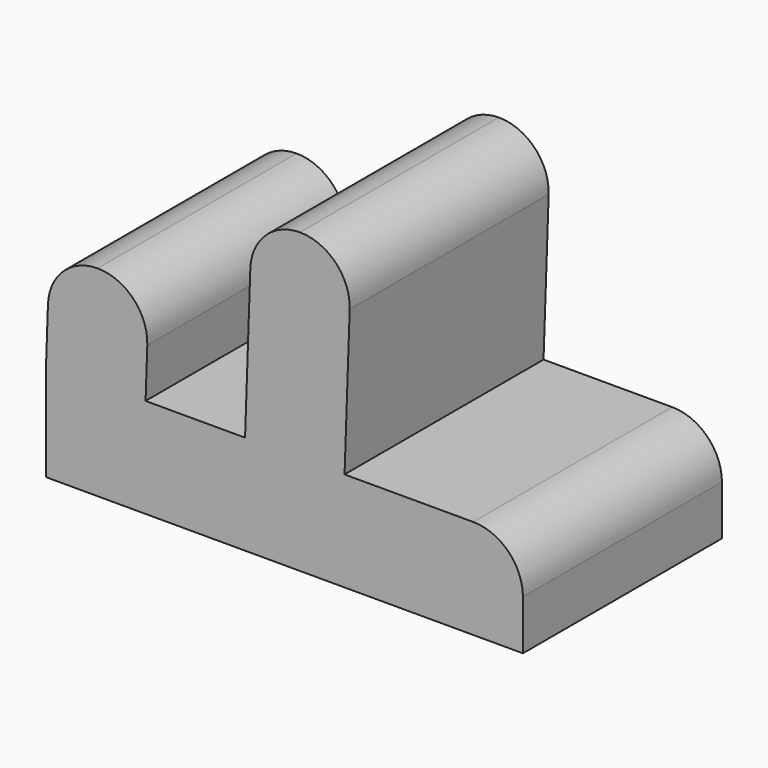
from build123d import *

# Parameters (mm, degrees)
F1_DEPTH    = 25
F2_R        = 5
F3_T1_DEPTH = 50.8882578448
F3_T3_DEPTH = 49.1422193702
F4_T1_DEPTH = 50.8882578448
F5_R        = 5


# Not quite as in the source:
# - a fillet or chamfer that OpenCascade refuses, or shapes differently, is made with other operations: its cross-section is extruded or revolved along the edge and cut away or added


with BuildPart() as f1:
    # F0 (on Front) → F1 (new body)
    with BuildSketch(Plane.XZ):
        Polygon((-29.6450223361, 14.0248785508), (-30, 3.8596482585), (-20, 3.8596482585), (-19.6450223361, 14.0248785508), align=None)
        Polygon((-20, 3.8596482585), (-30, 3.8596482585), (-30, -6.1403517415), (17.9300867021, -6.1403517415), (17.9300867021, 3.8596482585), (0, 3.8596482585), (-10, 3.8596482585), align=None)
        Polygon((-9.3028735371, 23.8227382193), (-10, 3.8596482585), (0, 3.8596482585), (0.6971264629, 23.8227382193), align=None)
    extrude(amount=F1_DEPTH)

    # F2
    f2_edges = [f1.edges().sort_by_distance(p)[0] for p in [
        (-29.645022, -12.5, 14.024879),
    ]]
    fillet(f2_edges, radius=F2_R)

    # F3: fillet of radius 5 on 2 edges, made by hand

    # F3_s2 → F3_t1 (cut)
    with BuildSketch(Plane.XZ.offset(-12.9441289224)):
        with BuildLine():
            ThreePointArc((-24.8226739051, 14.0248785508), (-21.2259749034, 12.4981704031), (-19.82571977, 8.8503810672))
            Line((-19.82571977, 8.8503810672), (-19.6450223361, 14.0248785508))
            Line((-19.6450223361, 14.0248785508), (-24.8226739051, 14.0248785508))
        make_face()
    extrude(amount=F3_T1_DEPTH, mode=Mode.SUBTRACT)

    # F3_s4 → F3_t3 (cut)
    with BuildSketch(Plane.XZ.offset(-12.0711096851)):
        with BuildLine():
            ThreePointArc((-9.4713837982, 18.9972357029), (-7.9477215154, 22.419437221), (-4.4744296631, 23.8227382193))
            Line((-4.4744296631, 23.8227382193), (-9.3028735371, 23.8227382193))
            Line((-9.3028735371, 23.8227382193), (-9.4713837982, 18.9972357029))
        make_face()
    extrude(amount=F3_T3_DEPTH, mode=Mode.SUBTRACT)

    # F4: fillet of radius 5 on 1 edges, made by hand

    # F4_s2 → F4_t1 (cut)
    with BuildSketch(Plane.XZ.offset(-12.9441289224)):
        with BuildLine():
            ThreePointArc((-4.4805251061, 23.8227382193), (-0.8838261044, 22.2960300716), (0.516429029, 18.6482407358))
            Line((0.516429029, 18.6482407358), (0.6971264629, 23.8227382193))
            Line((0.6971264629, 23.8227382193), (-4.4805251061, 23.8227382193))
        make_face()
    extrude(amount=F4_T1_DEPTH, mode=Mode.SUBTRACT)

    # F5
    f5_edges = [f1.edges().sort_by_distance(p)[0] for p in [
        (17.930087, -12.5, 3.859648),
    ]]
    fillet(f5_edges, radius=F5_R)


solid = f1.part
